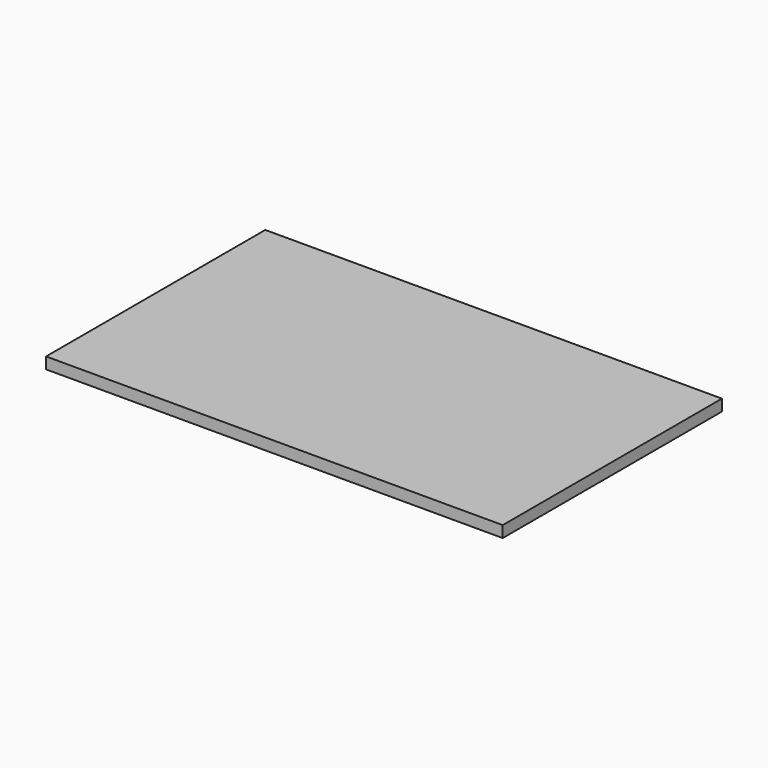
from build123d import *

# Parameters (mm, degrees)
F0_W            = 254
F0_H            = 152.4
F1_DEPTH        = 6.35
F5_COPIES_COUNT = 3


# Not quite as in the source:
# - a pattern or mirror of a feature is missing from the dataset's text; its kind, count and spacing are read off the source's solid


with BuildPart() as f1:
    # F0 (on Top) → F1 (new body)
    with BuildSketch(Plane.XY):
        Rectangle(F0_W, F0_H)
    extrude(amount=F1_DEPTH)

    # F4 (on face) → F5 (revolve)
    with BuildSketch(Plane.XZ.offset(-61.9125)):
        with BuildLine():
            Line((-71.4903970824, 0.7803010637), (-71.4903970824, -4.0456989363))
            ThreePointArc((-71.4903970824, -4.0456989363), (-68.0778997564, -2.6321962623), (-66.6643970824, 0.7803010637))
            Line((-66.6643970824, 0.7803010637), (-71.4903970824, 0.7803010637))
        make_face()
    f5 = revolve(axis=Axis((-71.4903970824, 61.9125, -1.6326989363), (0, 0, 1)))

    # F5_copies: F5 ×3 about axis
    f5_copies_axis = Axis((0, 20.6375, 0), (0, 0, 1))
    for i in range(1, F5_COPIES_COUNT):
        add(f5.rotate(f5_copies_axis, i * 360 / F5_COPIES_COUNT))


solid = f1.part
